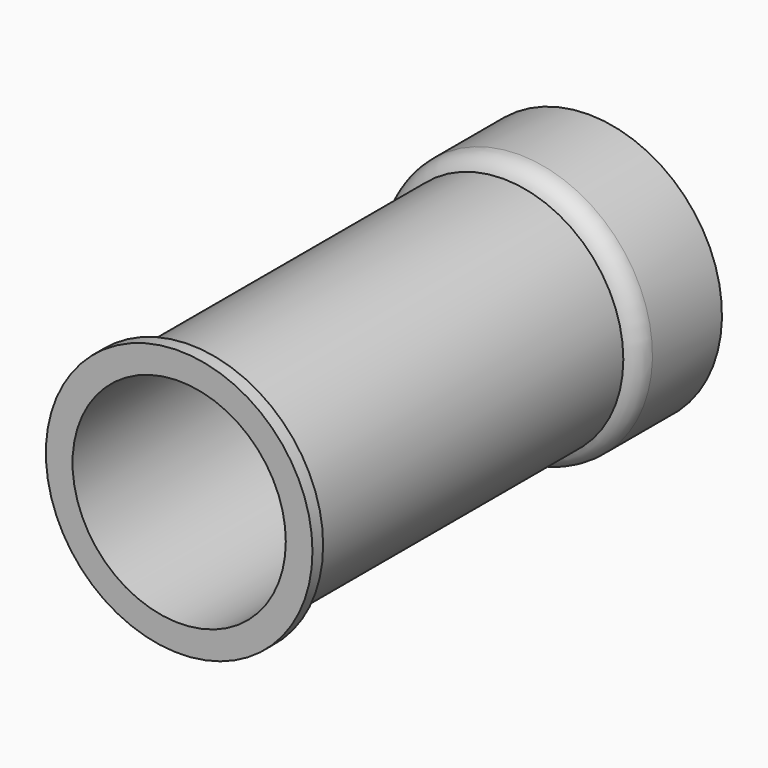
from build123d import *

# Parameters (mm, degrees)
F0_R     = 28.575
F0_R_2   = 25.4
F0_R_3   = 31.75
F3_DEPTH = 3.175


# Not quite as in the source:
# - a fillet or chamfer that OpenCascade refuses, or shapes differently, is made with other operations: its cross-section is extruded or revolved along the edge and cut away or added


with BuildPart() as f2:
    # F2: sweep along a path in F1
    with BuildLine(Plane.YZ) as f2_path:
        Line((0, 0), (101.6, 0))
    # F0 (on Front) → F2 (sweep)
    with BuildSketch(Plane.XZ):
        Circle(F0_R)
        Circle(F0_R_2, mode=Mode.SUBTRACT)
    sweep(path=f2_path.line)

    # F0 (on Front) → F3 (join)
    with BuildSketch(Plane.XZ):
        Circle(F0_R_3)
        Circle(F0_R, mode=Mode.SUBTRACT)
    extrude(amount=-F3_DEPTH)

    # F1 (on Right) → F4 (revolve)
    with BuildSketch(Plane.YZ):
        Polygon((96.52, 28.575), (101.6, 28.575), (121.92, 28.575), (121.92, 31.75), (96.52, 31.75), align=None)
    revolve(axis=Axis((0, 50.8, 0), (0, 1, 0)))

    # F5: fillet of radius 5.08 on 2 edges, made by hand

    # F5_s1 → F5_t2 (revolve, cut)
    with BuildSketch(Plane.XY):
        with BuildLine():
            ThreePointArc((28.575, 101.6), (26.2678865162, 99.7305202921), (25.4, 96.8907139607))
            Line((25.4, 96.8907139607), (25.4, 101.6))
            Line((25.4, 101.6), (28.575, 101.6))
        make_face()
    revolve(axis=Axis((0, 101.6, 0), (0, 1, 0)), mode=Mode.SUBTRACT)

    # F5_s3 → F5_t4 (revolve, cut)
    with BuildSketch(Plane.YZ):
        with BuildLine():
            ThreePointArc((96.52, 28.575), (98.3894797079, 30.8821134838), (101.2292860393, 31.75))
            Line((101.2292860393, 31.75), (96.52, 31.75))
            Line((96.52, 31.75), (96.52, 28.575))
        make_face()
    revolve(axis=Axis((0, 96.52, 0), (0, 1, 0)), mode=Mode.SUBTRACT)


solid = f2.part
